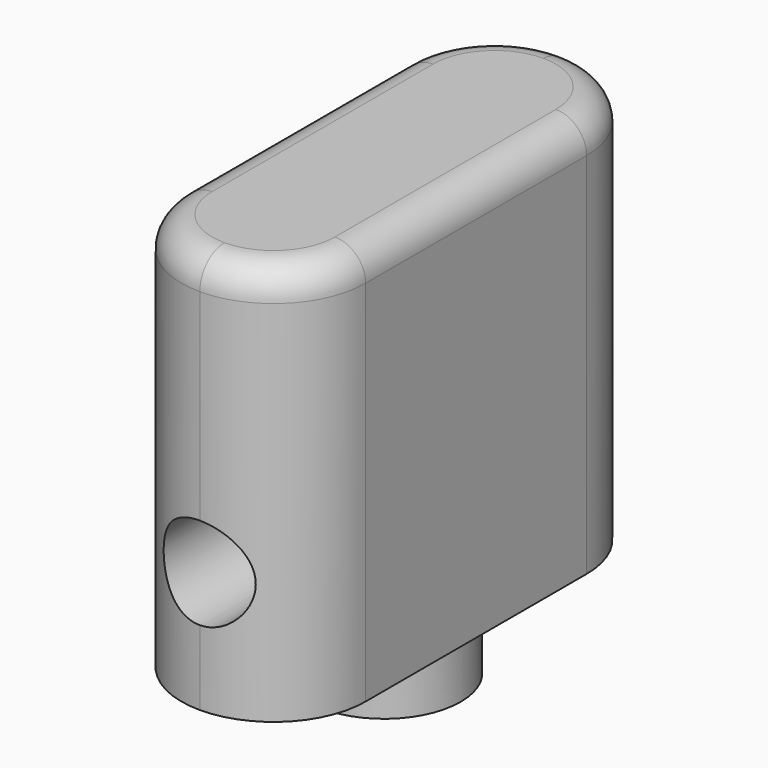
from build123d import *

# Parameters (mm, degrees)
F0_W     = 6
F0_H     = 15
F1_DEPTH = 13
F3_DEPTH = 2
F4_R     = 2.99999
F5_R     = 1
F6_R     = 1.5
F7_DEPTH = 10


# Not quite as in the source:
# - a fillet or chamfer is up to 0.001 mm smaller than in the source, because OpenCascade refuses the exact size


with BuildPart() as f1:
    # F0 (on Top) → F1 (new body)
    with BuildSketch(Plane.XY):
        with Locations((0, 7.5)):
            Rectangle(F0_W, F0_H)
    extrude(amount=F1_DEPTH)

    # F2 (on face) → F3 (join)
    with BuildSketch(Plane(origin=(0, 0, 0), x_dir=(1, 0, 0), z_dir=(0, 0, -1))):
        with BuildLine():
            ThreePointArc((-2.5, -7.5), (0, -10), (2.5, -7.5))
            Line((2.5, -7.5), (-2.5, -7.5))
        make_face()
        with BuildLine():
            Line((-2.5, -7.5), (2.5, -7.5))
            ThreePointArc((2.5, -7.5), (0, -5), (-2.5, -7.5))
        make_face()
    extrude(amount=F3_DEPTH)

    # F4 (radius 3 in the source; OpenCascade refuses exactly that, so slightly less here)
    f4_edges = [f1.edges().sort_by_distance(p)[0] for p in [
        (-3, 0, 6.5),
        (3, 0, 6.5),
        (3, 15, 6.5),
        (-3, 15, 6.5),
    ]]
    fillet(f4_edges, radius=F4_R)

    # F5
    f5_edges = [f1.edges().sort_by_distance(p)[0] for p in [
        (0, 15, 13),
        (2.121323, 14.121323, 13),
        (-2.121323, 14.121323, 13),
        (3, 7.5, 13),
        (-3, 7.5, 13),
        (2.121323, 0.878677, 13),
        (-2.121323, 0.878677, 13),
        (0, 0, 13),
    ]]
    fillet(f5_edges, radius=F5_R)

    # F6 (on Front) → F7 (cut)
    with BuildSketch(Plane.XZ):
        with Locations((0, 3.9348333655)):
            Circle(F6_R)
    extrude(amount=-F7_DEPTH, mode=Mode.SUBTRACT)


solid = f1.part
